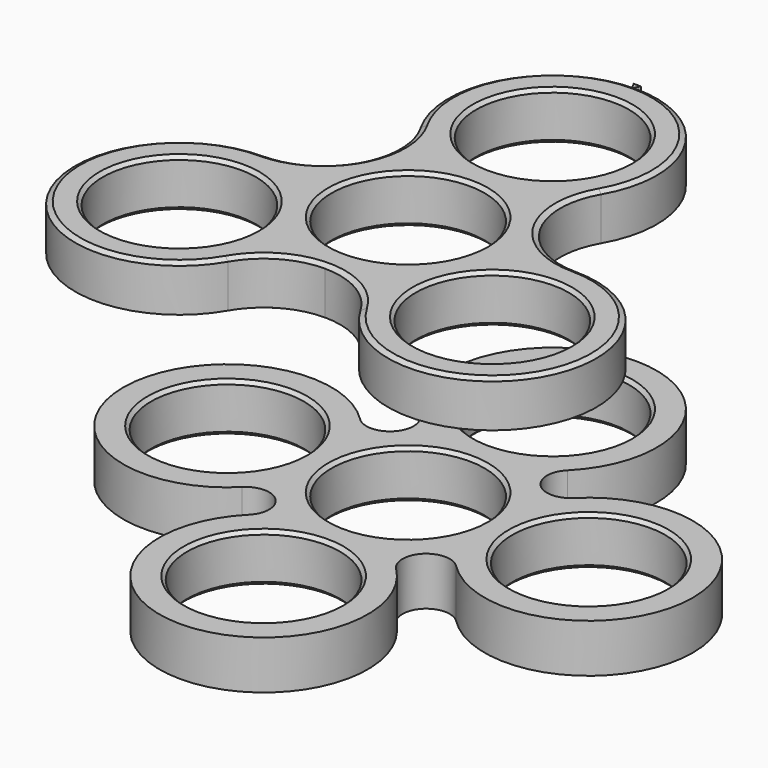
from build123d import *

# Parameters (mm, degrees)
F0_R         = 11.05
F1_DEPTH     = 7
F2_SIZE      = 0.5
F4_R         = 11.05
F5_DEPTH     = 7
F6_SIZE      = 0.5
F8_T2_ANGLE  = 120
F8_T4_ANGLE  = 120
F8_T6_ANGLE  = 240
F8_T8_ANGLE  = 120
F8_T10_ANGLE = 240
F8_T12_ANGLE = 120
F8_T14_ANGLE = 120
F8_T16_ANGLE = 240
F8_T18_ANGLE = 120
F8_T20_ANGLE = 240
F8_T22_ANGLE = 240
F8_T24_ANGLE = 240
F9_DEPTH     = 7


# Not quite as in the source:
# - a fillet or chamfer that OpenCascade refuses, or shapes differently, is made with other operations: its cross-section is extruded or revolved along the edge and cut away or added


with BuildPart() as f1:
    # F0 (on Top) → F1 (new body)
    with BuildSketch(Plane.XY):
        with BuildLine():
            ThreePointArc((13.033682327, 7.525), (11.5532630388, 13.05), (13.033682327, 18.575))
            ThreePointArc((13.033682327, 18.575), (0, 41.15), (-13.033682327, 18.575))
            ThreePointArc((-13.033682327, 18.575), (-11.5532630388, 13.05), (-13.033682327, 7.525))
            ThreePointArc((-13.033682327, 7.525), (-17.0782630388, 3.4804192882), (-22.6032630388, 2))
            ThreePointArc((-22.6032630388, 2), (-35.6369453657, -20.575), (-9.5695807118, -20.575))
            ThreePointArc((-9.5695807118, -20.575), (-5.525, -16.5304192882), (0, -15.05))
            ThreePointArc((0, -15.05), (5.525, -16.5304192882), (9.5695807118, -20.575))
            ThreePointArc((9.5695807118, -20.575), (35.6369453657, -20.575), (22.6032630388, 2))
            ThreePointArc((22.6032630388, 2), (17.0782630388, 3.4804192882), (13.033682327, 7.525))
        make_face()
        with Locations((-22.6032630388, -13.05)):
            Circle(F0_R, mode=Mode.SUBTRACT)
        with Locations((22.6032630388, -13.05)):
            Circle(F0_R, mode=Mode.SUBTRACT)
        Circle(F0_R, mode=Mode.SUBTRACT)
        with Locations((0, 26.1)):
            Circle(F0_R, mode=Mode.SUBTRACT)
    extrude(amount=F1_DEPTH)

    # F2
    f2_edges = [f1.edges().sort_by_distance(p)[0] for p in [
        (-11.553263, -13.05, 3.5),
        (-33.653263, -13.05, 0),
        (-33.653263, -13.05, 7),
        (11.05, 0, 3.5),
        (-11.05, 0, 0),
        (-11.05, 0, 7),
        (11.05, 26.1, 3.5),
        (-11.05, 26.1, 0),
        (-11.05, 26.1, 7),
        (33.653263, -13.05, 3.5),
        (11.553263, -13.05, 0),
        (11.553263, -13.05, 7),
    ]]
    chamfer(f2_edges, length=F2_SIZE)

    # F8: chamfer of 0.75 x 0.3904252879 on 10 edges, made by hand

    # F8_s1 → F8_t2 (revolve, cut)
    with BuildSketch(Plane.YZ.offset(22.6032630388)):
        Polygon((1.25, 0), (2, 0.3904252879), (2, 0), align=None)
    revolve(axis=Axis((22.6032630388, 13.05, 0), (0, 0, -1)), revolution_arc=F8_T2_ANGLE, mode=Mode.SUBTRACT)

    # F8_s3 → F8_t4 (revolve, cut)
    with BuildSketch(Plane(origin=(-11.3016315194, 19.575, 0), x_dir=(0, 0, 1), z_dir=(-0.5, 0.8660254038, 0))):
        Polygon((0, -1.25), (0.3904252879, -2), (0, -2), align=None)
    revolve(axis=Axis((-22.6032630388, 13.05, 0), (0, 0, -1)), revolution_arc=F8_T4_ANGLE, mode=Mode.SUBTRACT)

    # F8_s5 → F8_t6 (revolve, cut)
    with BuildSketch(Plane.YZ.offset(-22.6032630388)):
        Polygon((1.25, 0), (2, 0.3904252879), (2, 0), align=None)
    revolve(axis=Axis((-22.6032630388, -13.05, 0), (0, 0, 1)), revolution_arc=F8_T6_ANGLE, mode=Mode.SUBTRACT)

    # F8_s7 → F8_t8 (revolve, cut)
    with BuildSketch(Plane(origin=(-11.3016315194, -19.575, 0), x_dir=(0, 0, 1), z_dir=(-0.5, -0.8660254038, 0))):
        Polygon((0, -1.25), (0.3904252879, -2), (0, -2), align=None)
    revolve(axis=Axis((0, -26.1, 0), (0, 0, -1)), revolution_arc=F8_T8_ANGLE, mode=Mode.SUBTRACT)

    # F8_s9 → F8_t10 (revolve, cut)
    with BuildSketch(Plane(origin=(11.3016315194, -19.575, 0), x_dir=(0, 0, 1), z_dir=(-0.5, 0.8660254038, 0))):
        Polygon((0, -1.25), (0.3904252879, -2), (0, -2), align=None)
    revolve(axis=Axis((22.6032630388, -13.05, 0), (0, 0, 1)), revolution_arc=F8_T10_ANGLE, mode=Mode.SUBTRACT)

    # F8_s11 → F8_t12 (revolve, cut)
    with BuildSketch(Plane(origin=(11.3016315194, 19.575, 0), x_dir=(0, 0, 1), z_dir=(0.5, 0.8660254038, 0))):
        Polygon((6.6095747121, 2), (7, 1.25), (7, 2), align=None)
    revolve(axis=Axis((22.6032630388, 13.05, 7), (0, 0, 1)), revolution_arc=F8_T12_ANGLE, mode=Mode.SUBTRACT)

    # F8_s13 → F8_t14 (revolve, cut)
    with BuildSketch(Plane.YZ.offset(-22.6032630388)):
        Polygon((2, 6.6095747121), (1.25, 7), (2, 7), align=None)
    revolve(axis=Axis((-22.6032630388, 13.05, 7), (0, 0, 1)), revolution_arc=F8_T14_ANGLE, mode=Mode.SUBTRACT)

    # F8_s15 → F8_t16 (revolve, cut)
    with BuildSketch(Plane.YZ.offset(-22.6032630388)):
        Polygon((2, 6.6095747121), (1.25, 7), (2, 7), align=None)
    revolve(axis=Axis((-22.6032630388, -13.05, 7), (0, 0, 1)), revolution_arc=F8_T16_ANGLE, mode=Mode.SUBTRACT)

    # F8_s17 → F8_t18 (revolve, cut)
    with BuildSketch(Plane(origin=(11.3016315194, -19.575, 0), x_dir=(0, 0, 1), z_dir=(0.5, -0.8660254038, 0))):
        Polygon((6.6095747121, 2), (7, 1.25), (7, 2), align=None)
    revolve(axis=Axis((0, -26.1, 7), (0, 0, 1)), revolution_arc=F8_T18_ANGLE, mode=Mode.SUBTRACT)

    # F8_s19 → F8_t20 (revolve, cut)
    with BuildSketch(Plane(origin=(11.3016315194, -19.575, 0), x_dir=(0, 0, 1), z_dir=(-0.5, 0.8660254038, 0))):
        Polygon((6.6095747121, -2), (7, -1.25), (7, -2), align=None)
    revolve(axis=Axis((22.6032630388, -13.05, 7), (0, 0, 1)), revolution_arc=F8_T20_ANGLE, mode=Mode.SUBTRACT)

    # F8_s21 → F8_t22 (revolve, cut)
    with BuildSketch(Plane(origin=(11.3016315194, 19.575, 0), x_dir=(0, 0, 1), z_dir=(-0.5, -0.8660254038, 0))):
        Polygon((6.6095747121, -2), (7, -1.25), (7, -2), align=None)
    revolve(axis=Axis((0, 26.1, 7), (0, 0, 1)), revolution_arc=F8_T22_ANGLE, mode=Mode.SUBTRACT)

    # F8_s23 → F8_t24 (revolve, cut)
    with BuildSketch(Plane(origin=(11.3016315194, 19.575, 0), x_dir=(0, 0, 1), z_dir=(-0.5, -0.8660254038, 0))):
        Polygon((0, -1.25), (0.3904252879, -2), (0, -2), align=None)
    revolve(axis=Axis((0, 26.1, 0), (0, 0, 1)), revolution_arc=F8_T24_ANGLE, mode=Mode.SUBTRACT)


with BuildPart() as f5:
    # F4 (on offset) → F5 (new body)
    with BuildSketch(Plane(origin=(0, 0, -35), x_dir=(1, 0, 0), z_dir=(0, 0, -1))):
        with BuildLine():
            ThreePointArc((15.4580429431, 10.6419570569), (10.6419570569, 10.6419570569), (10.6419570569, 15.4580429431))
            ThreePointArc((10.6419570569, 15.4580429431), (0, 41.15), (-10.6419570569, 15.4580429431))
            ThreePointArc((-10.6419570569, 15.4580429431), (-10.6419570569, 10.6419570569), (-15.4580429431, 10.6419570569))
            ThreePointArc((-15.4580429431, 10.6419570569), (-41.15, 0), (-15.4580429431, -10.6419570569))
            ThreePointArc((-15.4580429431, -10.6419570569), (-10.6419570569, -10.6419570569), (-10.6419570569, -15.4580429431))
            ThreePointArc((-10.6419570569, -15.4580429431), (0, -41.15), (10.6419570569, -15.4580429431))
            ThreePointArc((10.6419570569, -15.4580429431), (10.6419570569, -10.6419570569), (15.4580429431, -10.6419570569))
            ThreePointArc((15.4580429431, -10.6419570569), (41.15, 0), (15.4580429431, 10.6419570569))
        make_face()
        with Locations((0, -26.1)):
            Circle(F4_R, mode=Mode.SUBTRACT)
        with Locations((-26.1, 0)):
            Circle(F4_R, mode=Mode.SUBTRACT)
        Circle(F4_R, mode=Mode.SUBTRACT)
        with Locations((0, 26.1)):
            Circle(F4_R, mode=Mode.SUBTRACT)
        with Locations((26.1, 0)):
            Circle(F4_R, mode=Mode.SUBTRACT)
    extrude(amount=-F5_DEPTH)

    # F6
    f6_edges = [f5.edges().sort_by_distance(p)[0] for p in [
        (-15.05, 0, -31.5),
        (-37.15, 0, -35),
        (-37.15, 0, -28),
        (11.05, 0, -31.5),
        (-11.05, 0, -35),
        (-11.05, 0, -28),
        (11.05, 26.1, -31.5),
        (-11.05, 26.1, -35),
        (-11.05, 26.1, -28),
        (37.15, 0, -31.5),
        (15.05, 0, -35),
        (15.05, 0, -28),
        (11.05, -26.1, -31.5),
        (-11.05, -26.1, -35),
        (-11.05, -26.1, -28),
    ]]
    chamfer(f6_edges, length=F6_SIZE)


with BuildPart() as f9:
    # F7 (on face) → F9 (new body, through all)
    with BuildSketch(Plane.XY.offset(7)):
        with BuildLine():
            Line((-0.3878236262, 41.1450022544), (0, 40.4))
            Line((0, 40.4), (0.3878236262, 41.1450022544))
            ThreePointArc((0.3878236262, 41.1450022544), (0, 41.15), (-0.3878236262, 41.1450022544))
        make_face()
        with BuildLine():
            ThreePointArc((-0.3878236262, 41.1450022544), (0, 41.15), (0.3878236262, 41.1450022544))
            Line((0.3878236262, 41.1450022544), (0.5205670506, 41.4))
            Line((0.5205670506, 41.4), (-0.5205670506, 41.4))
            Line((-0.5205670506, 41.4), (-0.3878236262, 41.1450022544))
        make_face()
    extrude(amount=-F9_DEPTH)


solid = Compound([f1.part, f5.part, f9.part])
